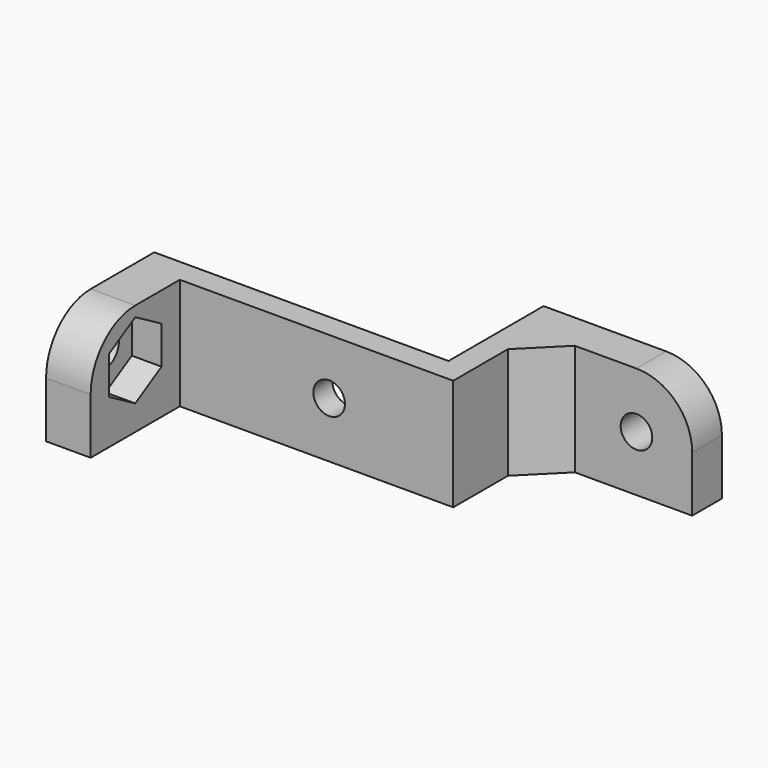
from build123d import *

# Parameters (mm, degrees)
F1_DEPTH = 15
F2_R     = 2.125
F3_DEPTH = 25
F4_SIZE  = 5
F5_R     = 7.5
F6_R     = 2.25
F7_DEPTH = 25
F9_DEPTH = 4


# Not quite as in the source:
# - a feature names something its author has since deleted; it is built from what else it names


with BuildPart() as f1:
    # F0 (on Top) → F1 (new body)
    with BuildSketch(Plane.XY):
        Polygon((-16.7, 0), (0, 0), (16.7, 0), (16.7, 14.2), (37.5, 14.2), (37.5, 19.2), (13.5, 19.2), (13.5, 3.2), (0, 3.2), (-13.5, 3.2), (-26.1, 3.2), (-26.1, -15), (-20.1, -15), (-20.1, 0), align=None)
    extrude(amount=F1_DEPTH)

    # F2 (on face) → F3 (cut)
    with BuildSketch(Plane.XZ):
        with Locations((0, 7.5)):
            Circle(F2_R)
        with Locations((30, 7.5)):
            Circle(F2_R)
    extrude(amount=-F3_DEPTH, mode=Mode.SUBTRACT)

    # F4
    f4_edges = [f1.edges().sort_by_distance(p)[0] for p in [
        (16.7, 14.2, 7.5),
    ]]
    chamfer(f4_edges, length=F4_SIZE)

    # F5
    f5_edges = [f1.edges().sort_by_distance(p)[0] for p in [
        (37.5, 16.7, 15),
        (-23.1, -15, 15),
    ]]
    fillet(f5_edges, radius=F5_R)

    # F6 (on face) → F7 (cut)
    with BuildSketch(Plane.YZ.offset(-20.1)):
        with Locations((-7.5, 8.5048094716)):
            Circle(F6_R)
    extrude(amount=-F7_DEPTH, mode=Mode.SUBTRACT)

    # F8 (on face) → F9 (cut)
    with BuildSketch(Plane.YZ.offset(-20.1)):
        Polygon((-3.0775, 5.9514779061), (-3.0775, 11.0581410371), (-7.5, 13.6114726026), (-11.9225, 11.0581410371), (-11.9225, 5.9514779061), (-7.5, 3.3981463406), align=None)
    extrude(amount=-F9_DEPTH, mode=Mode.SUBTRACT)


solid = f1.part
